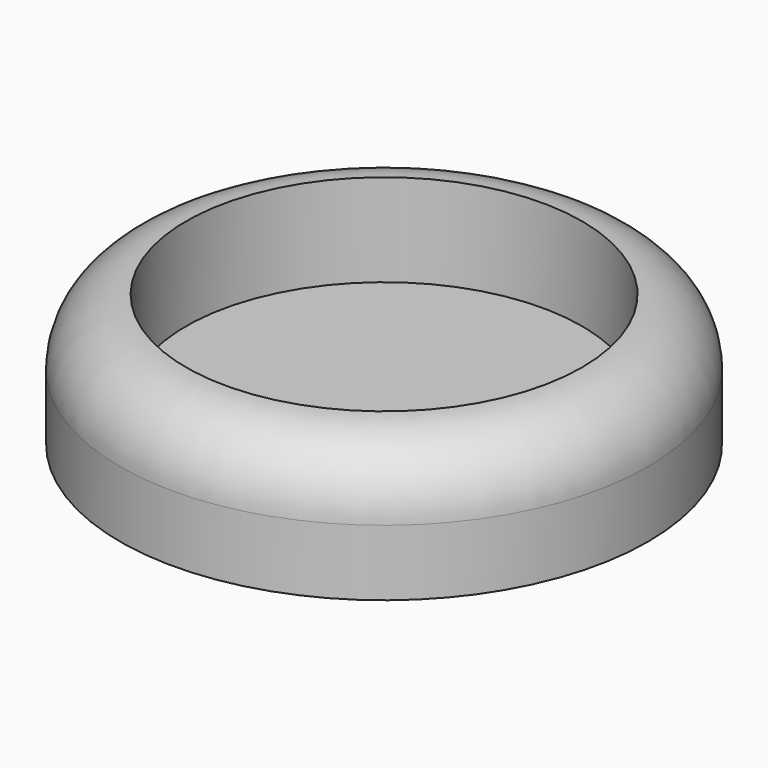
from build123d import *

# Parameters (mm, degrees)
F0_R     = 20
F0_R_2   = 15
F1_DEPTH = 7
F2_R     = 20
F3_DEPTH = 3
F4_R     = 4.99999


# Not quite as in the source:
# - a fillet or chamfer is up to 0.001 mm smaller than in the source, because OpenCascade refuses the exact size


with BuildPart() as f1:
    # F0 (on Top) → F1 (new body)
    with BuildSketch(Plane.XY):
        Circle(F0_R)
        Circle(F0_R_2, mode=Mode.SUBTRACT)
    extrude(amount=F1_DEPTH)

    # F2 (on Top) → F3 (join)
    with BuildSketch(Plane.XY):
        Circle(F2_R)
    extrude(amount=-F3_DEPTH)

    # F4 (radius 5 in the source; OpenCascade refuses exactly that, so slightly less here)
    f4_edges = [f1.edges().sort_by_distance(p)[0] for p in [
        (-20, 0, 7),
    ]]
    fillet(f4_edges, radius=F4_R)


solid = f1.part
